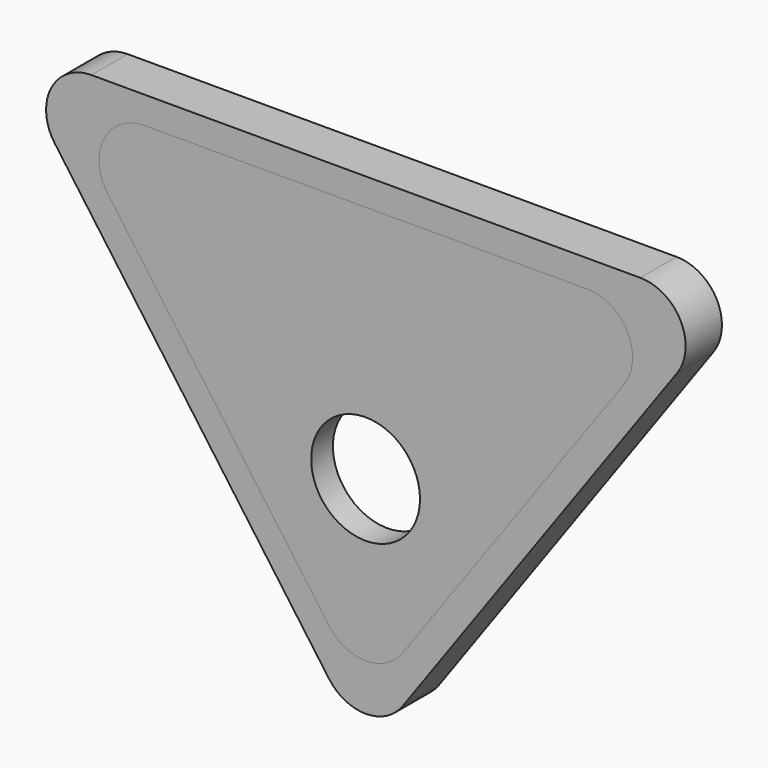
from build123d import *

# Parameters (mm, degrees)
F2_DEPTH = 5
F0_R     = 6
F3_DEPTH = 3


# Not quite as in the source:
# - the program builds the solid bodies; features that only make, move or delete a surface that nothing else refers to are left out


with BuildPart() as f2:
    # F0 (on Front) → F2 (new body)
    with BuildSketch(Plane.XZ):
        with BuildLine():
            ThreePointArc((-5.6796433529, -7.9150359145), (-5.293653969, -2.716929652), (-9.7419783486, 0))
            Line((-9.7419783486, 0), (-70.2580216514, 0))
            ThreePointArc((-70.2580216514, 0), (-74.706346031, -2.716929652), (-74.3203566471, -7.9150359145))
            Line((-74.3203566471, -7.9150359145), (-44.0623349957, -50.0820019003))
            ThreePointArc((-44.0623349957, -50.0820019003), (-40, -52.1669659858), (-35.9376650043, -50.0820019003))
            Line((-35.9376650043, -50.0820019003), (-5.6796433529, -7.9150359145))
        make_face()
        with BuildLine():
            ThreePointArc((-15.5871653577, -3), (-11.1388409781, -5.716929652), (-11.524830362, -10.9150359145))
            Line((-11.524830362, -10.9150359145), (-35.9376650043, -44.9362677002))
            ThreePointArc((-35.9376650043, -44.9362677002), (-40, -47.0212317857), (-44.0623349957, -44.9362677002))
            Line((-44.0623349957, -44.9362677002), (-68.475169638, -10.9150359145))
            ThreePointArc((-68.475169638, -10.9150359145), (-68.8611590219, -5.716929652), (-64.4128346423, -3))
            Line((-64.4128346423, -3), (-15.5871653577, -3))
        make_face(mode=Mode.SUBTRACT)
    extrude(amount=-F2_DEPTH)


with BuildPart() as f3:
    # F0 (on Front) → F3 (new body)
    with BuildSketch(Plane.XZ):
        with BuildLine():
            Line((-35.9376650043, -44.9362677002), (-11.524830362, -10.9150359145))
            ThreePointArc((-11.524830362, -10.9150359145), (-11.1388409781, -5.716929652), (-15.5871653577, -3))
            Line((-15.5871653577, -3), (-64.4128346423, -3))
            ThreePointArc((-64.4128346423, -3), (-68.8611590219, -5.716929652), (-68.475169638, -10.9150359145))
            Line((-68.475169638, -10.9150359145), (-44.0623349957, -44.9362677002))
            ThreePointArc((-44.0623349957, -44.9362677002), (-40, -47.0212317857), (-35.9376650043, -44.9362677002))
        make_face()
        with Locations((-40.0314554572, -29.3799452484)):
            Circle(F0_R, mode=Mode.SUBTRACT)
    extrude(amount=-F3_DEPTH)


solid = Compound([f2.part, f3.part])
